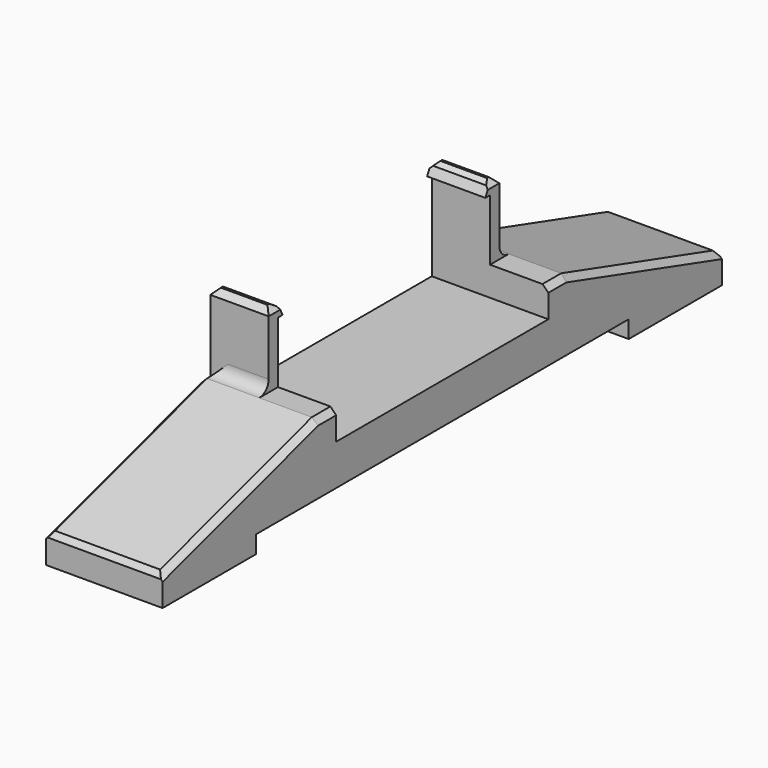
from build123d import *

# Parameters (mm, degrees)
F1_DEPTH     = 10
F3_DEPTH     = 10
F4_T1_DEPTH  = 15.1433659759
F4_T3_DEPTH  = 7.1433659759
F4_T5_DEPTH  = 13.2619951725
F4_T7_DEPTH  = 7.1433659759
F4_T9_DEPTH  = 41.6647551639
F4_T11_DEPTH = 23.8798106503
F4_T13_DEPTH = 10.9435440675
F4_T15_DEPTH = 41.6647551639
F4_T17_DEPTH = 10.9435440675
F4_T19_DEPTH = 6.3718610795
F4_T21_DEPTH = 6.3718610795
F4_T26_DEPTH = 41.6647551639
F4_T31_DEPTH = 41.6647551639
F5_R         = 1.99999


# Not quite as in the source:
# - a fillet or chamfer that OpenCascade refuses, or shapes differently, is made with other operations: its cross-section is extruded or revolved along the edge and cut away or added
# - a fillet or chamfer is up to 0.001 mm smaller than in the source, because OpenCascade refuses the exact size


with BuildPart() as f1:
    # F0 (on Right) → F1 (new body)
    with BuildSketch(Plane.YZ):
        Polygon((22.75, 10), (-22.75, 10), (-22.75, 15), (-24.75, 15), (-26.75, 15), (-60, 5), (-60, 0), (-40, 0), (-40, 3), (40, 3), (40, 0), (60, 0), (60, 5), (26.75, 15), (24.75, 15), (22.75, 15), align=None)
        Polygon((-24.75, 15), (-22.75, 15), (-22.75, 25.5), (-21.75, 25.5), (-22.75, 27.5), (-24.75, 27.5), align=None)
        Polygon((22.75, 25.5), (22.75, 15), (24.75, 15), (24.75, 27.5), (22.75, 27.5), (21.75, 25.5), align=None)
    extrude(amount=F1_DEPTH)

    # F2 (on face) → F3 (join)
    with BuildSketch(Plane.YZ.offset(10)):
        Polygon((-22.75, 15), (-24.75, 15), (-26.75, 15), (-60, 5), (-60, 0), (-40, 0), (-40, 3), (40, 3), (40, 0), (60, 0), (60, 5), (26.75, 15), (24.75, 15), (22.75, 15), (22.75, 10), (-22.75, 10), align=None)
    extrude(amount=F3_DEPTH)

    # F4: chamfer of 1 on 18 edges, made by hand

    # F4_s2 → F4_t1 (cut)
    with BuildSketch(Plane.YZ.offset(-2.571682988)):
        Polygon((-24.75, 26.5), (-23.75, 27.5), (-24.75, 27.5), align=None)
        Polygon((23.75, 27.5), (24.75, 26.5), (24.75, 27.5), align=None)
    extrude(amount=F4_T1_DEPTH, mode=Mode.SUBTRACT)

    # F4_s4 → F4_t3 (cut)
    with BuildSketch(Plane.XZ.offset(20.178317012)):
        Polygon((10, 26.5), (9, 27.5), (10, 27.5), align=None)
        Polygon((0, 26.5), (1, 27.5), (0, 27.5), align=None)
    extrude(amount=F4_T3_DEPTH, mode=Mode.SUBTRACT)

    # F4_s6 → F4_t5 (cut)
    with BuildSketch(Plane.YZ.offset(-1.6309975863)):
        Polygon((-23.3680339887, 27.5), (-22.4736067977, 26.9472135955), (-22.75, 27.5), align=None)
        Polygon((22.4736067977, 26.9472135955), (23.3680339887, 27.5), (22.75, 27.5), align=None)
    extrude(amount=F4_T5_DEPTH, mode=Mode.SUBTRACT)

    # F4_s8 → F4_t7 (cut)
    with BuildSketch(Plane.XZ.offset(-27.321682988)):
        Polygon((10, 26.5), (9, 27.5), (10, 27.5), align=None)
        Polygon((0, 26.5), (1, 27.5), (0, 27.5), align=None)
    extrude(amount=F4_T7_DEPTH, mode=Mode.SUBTRACT)

    # F4_s10 → F4_t9 (cut)
    with BuildSketch(Plane(origin=(0, 56.1067611738, -16.8742138869), x_dir=(1, 0, 0), z_dir=(0, -0.9576278865, 0.2880083869))):
        Polygon((19, 22.0686426482), (20, 21.0686426482), (20, 22.0686426482), align=None)
    extrude(amount=F4_T9_DEPTH, mode=Mode.SUBTRACT)

    # F4_s12 → F4_t11 (cut)
    with BuildSketch(Plane.YZ.offset(-1.9399053251)):
        Polygon((59.2880083869, 5.214132816), (60, 4.2565049294), (60, 5), align=None)
        Polygon((-60, 4.2565049294), (-59.2880083869, 5.214132816), (-60, 5), align=None)
    extrude(amount=F4_T11_DEPTH, mode=Mode.SUBTRACT)

    # F4_s14 → F4_t13 (cut)
    with BuildSketch(Plane.XZ.offset(-31.1218610795)):
        Polygon((19, 15), (20, 14), (20, 15), align=None)
    extrude(amount=F4_T13_DEPTH, mode=Mode.SUBTRACT)

    # F4_s16 → F4_t15 (cut)
    with BuildSketch(Plane(origin=(0, -16.2074297434, -4.8744149604), x_dir=(1, 0, 0), z_dir=(0, -0.9576278865, -0.2880083869))):
        Polygon((19, 22.0686426482), (20, 21.0686426482), (20, 22.0686426482), align=None)
    extrude(amount=F4_T15_DEPTH, mode=Mode.SUBTRACT)

    # F4_s18 → F4_t17 (cut)
    with BuildSketch(Plane.XZ.offset(20.178317012)):
        Polygon((19, 15), (20, 14), (20, 15), align=None)
    extrude(amount=F4_T17_DEPTH, mode=Mode.SUBTRACT)

    # F4_s20 → F4_t19 (cut)
    with BuildSketch(Plane.XZ.offset(24.75)):
        Polygon((0, 14), (1, 15), (0, 15), align=None)
    extrude(amount=F4_T19_DEPTH, mode=Mode.SUBTRACT)

    # F4_s22 → F4_t21 (cut)
    with BuildSketch(Plane.XZ.offset(-31.1218610795)):
        Polygon((0, 14), (1, 15), (0, 15), align=None)
    extrude(amount=F4_T21_DEPTH, mode=Mode.SUBTRACT)


with BuildPart() as f4_tool24:
    # F4_s25 → F4_t26 (new body)
    with BuildSketch(Plane(origin=(0, -16.2074297434, -4.8744149604), x_dir=(1, 0, 0), z_dir=(0, -0.9576278865, -0.2880083869))):
        Polygon((0, 21.0686426482), (1, 22.0686426482), (0, 22.0686426482), align=None)
    extrude(amount=F4_T26_DEPTH)

    split(bisect_by=Plane.XZ.offset(24.75), keep=Keep.TOP)


with BuildPart() as f1_1:
    add(f1.part)

    # F4_t23: cut F4_tool24
    add(f4_tool24.part, mode=Mode.SUBTRACT)


with BuildPart() as f4_tool29:
    # F4_s30 → F4_t31 (new body)
    with BuildSketch(Plane(origin=(0, 56.1067611738, -16.8742138869), x_dir=(1, 0, 0), z_dir=(0, -0.9576278865, 0.2880083869))):
        Polygon((0, 21.0686426482), (1, 22.0686426482), (0, 22.0686426482), align=None)
    extrude(amount=F4_T31_DEPTH)

    split(bisect_by=Plane.XZ.offset(-24.75), keep=Keep.BOTTOM)


with BuildPart() as f1_2:
    add(f1_1.part)

    # F4_t28: cut F4_tool29
    add(f4_tool29.part, mode=Mode.SUBTRACT)

    # F5 (radius 2 in the source; OpenCascade refuses exactly that, so slightly less here)
    f5_edges = [f1_2.edges().sort_by_distance(p)[0] for p in [
        (5.5, -24.75, 15),
        (5.5, 24.75, 15),
    ]]
    fillet(f5_edges, radius=F5_R)


solid = f1_2.part
